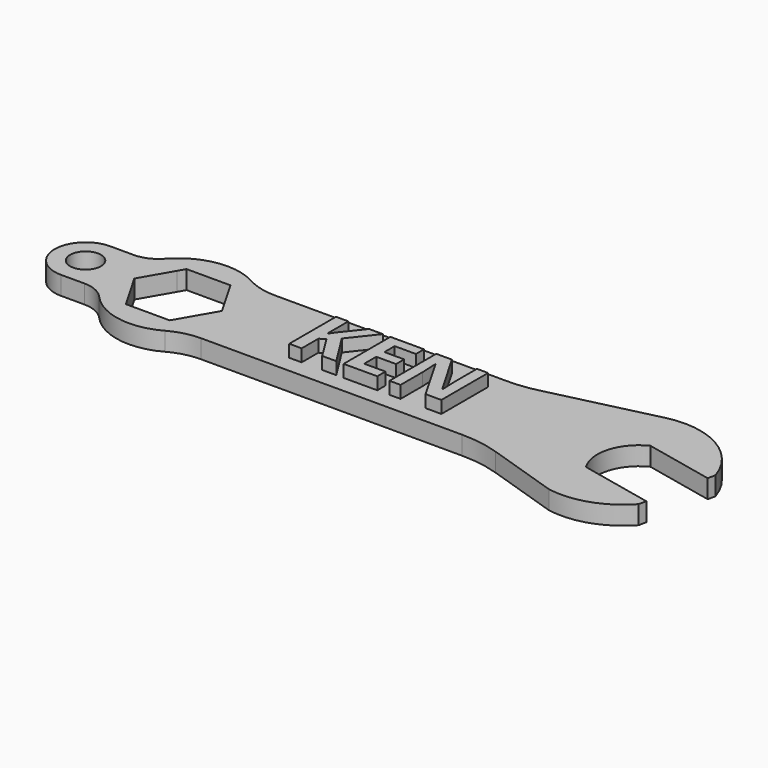
from build123d import *

# Parameters (mm, degrees)
F1_DEPTH     = 3
F2_TEXT_SIZE = 13.2673814531
F3_DEPTH     = 2
F4_R         = 2.5
F5_DEPTH     = 3


# Not quite as in the source:
# - a feature names something its author has since deleted; it is built from what else it names
# - Text() gives the source's letters only with a copy of the font that has no kerning and outlines rounded to 1/6400 em; it was checked with that copy


with BuildPart() as f1:
    # F0 (on Top) → F1 (new body)
    with BuildSketch(Plane.XY):
        with BuildLine():
            ThreePointArc((12.6289075872, 8.0475489588), (10.3210728444, 7.6373589266), (7.9810964369, 7.5))
            Line((7.9810964369, 7.5), (-29.6682382471, 7.5))
            ThreePointArc((-29.6682382471, 7.5), (-32.1682382471, 7.8175416345), (-34.5094674298, 8.75))
            ThreePointArc((-34.5094674298, 8.75), (-41.0213663649, 9.859455491), (-46.8042565376, 6.6666666667))
            ThreePointArc((-46.8042565376, 6.6666666667), (-48.4897950478, 5.4356453541), (-50.5310365001, 5))
            Line((-50.5310365001, 5), (-54.3506966126, 5))
            ThreePointArc((-54.3506966126, 5), (-57.8862305185, 3.5355339059), (-59.3506966126, 0))
            ThreePointArc((-59.3506966126, 0), (-57.8862305185, -3.5355339059), (-54.3506966126, -5))
            Line((-54.3506966126, -5), (-50.5310365001, -5))
            ThreePointArc((-50.5310365001, -5), (-48.4897950478, -5.4356453541), (-46.8042565376, -6.6666666667))
            ThreePointArc((-46.8042565376, -6.6666666667), (-41.0213663649, -9.859455491), (-34.5094674298, -8.75))
            ThreePointArc((-34.5094674298, -8.75), (-32.1682382471, -7.8175416345), (-29.6682382471, -7.5))
            Line((-29.6682382471, -7.5), (12.6678347331, -7.5))
            ThreePointArc((12.6678347331, -7.5), (15.812651654, -7.7487943018), (18.8792273218, -8.4889873466))
            Line((18.8792273218, -8.4889873466), (30.5844321556, -12.3133823895))
            ThreePointArc((30.5844321556, -12.3133823895), (36.7798399636, -11.827930201), (41.9758511797, -8.4190874096))
            Line((41.9758511797, -8.4190874096), (42.2432588852, -7.1816752039))
            Line((42.2432588852, -7.1816752039), (30.4154777171, -4.6256637076))
            ThreePointArc((30.4154777171, -4.6256637076), (29.6442094298, 0.8026234887), (33.156330505, 5.0128683997))
            Line((33.156330505, 5.0128683997), (44.3555236847, 2.592696255))
            Line((44.3555236847, 2.592696255), (44.6277974258, 3.852625732))
            ThreePointArc((44.6277974258, 3.852625732), (38.8546217522, 10.9002918904), (29.831436366, 12.1577819008))
            Line((29.831436366, 12.1577819008), (12.6289075872, 8.0475489588))
        make_face()
        Polygon((-43.5657825452, 5), (-42.9016152519, 6.1503714968), (-35.7997779733, 6.1503714968), (-32.2488593341, 0), (-35.7997779733, -6.1503714968), (-42.9016152519, -6.1503714968), (-43.5657825452, -5), (-46.4525338911, 0), align=None, mode=Mode.SUBTRACT)
    extrude(amount=F1_DEPTH)

    # F2 (on face) → F3 (join)
    with BuildSketch(Plane.XY.offset(3)):
        with Locations((-18.7758425309, -4.7129575396)):
            Text('KEN', F2_TEXT_SIZE, font='Open Sans', font_style=FontStyle.BOLD, text_align=(TextAlign.LEFT, TextAlign.BOTTOM))
    extrude(amount=F3_DEPTH)

    # F4 (on face) → F5 (cut, through all)
    with BuildSketch(Plane.XY.offset(3)):
        with Locations((-54.3506966126, 0)):
            Circle(F4_R)
    extrude(amount=-F5_DEPTH, mode=Mode.SUBTRACT)


solid = f1.part
